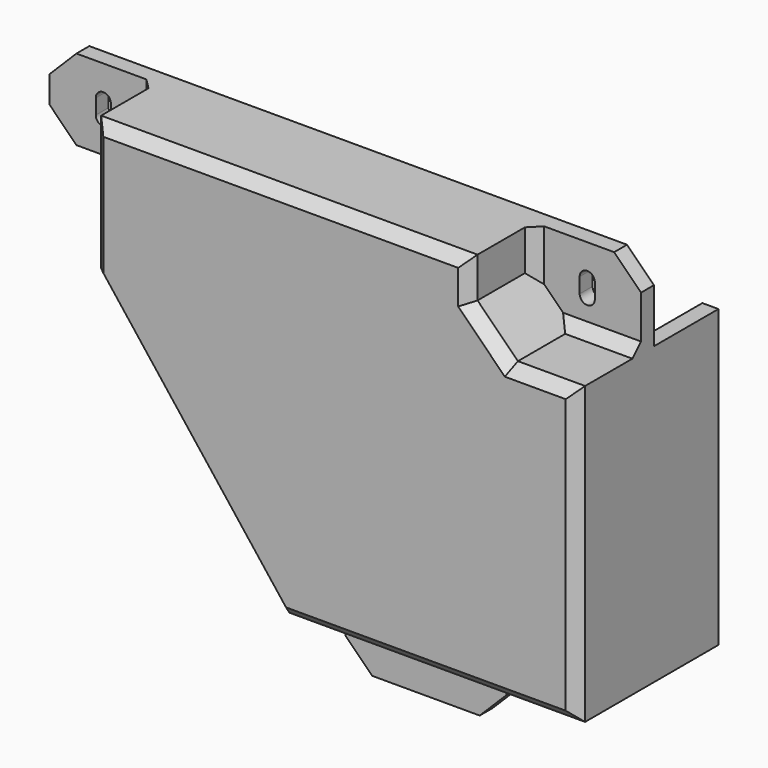
from build123d import *

# Parameters (mm, degrees)
F0_W      = 279.4
F0_H      = 213.36
F1_DEPTH  = 83.82
F2_W      = 76.2
F2_H      = 35.56
F2_W_2    = 50.8
F2_H_2    = 38.1
F3_DEPTH  = 38.1
F2_W_3    = 63.5
F4_DEPTH  = 83.82
F5_T      = -7.62
F6_W      = 38.1
F6_H      = 38.1
F6_H_2    = 35.56
F7_DEPTH  = 341.884
F9_DEPTH  = 7.62
F10_SIZE  = 5.08
F11_W     = 84.455
F11_H     = 38.1
F12_DEPTH = 25.4
F13_W     = 15.24
F13_H     = 12.7
F14_DEPTH = 12.7


# Not quite as in the source:
# - a feature names something its author has since deleted; it is built from what else it names


with BuildPart() as f1:
    # F0 (on Front) → F1 (new body)
    with BuildSketch(Plane.XZ):
        with Locations((-139.7, 106.68)):
            Rectangle(F0_W, F0_H)
    extrude(amount=F1_DEPTH)

    # F2 (on face) → F3 (cut)
    with BuildSketch(Plane.XZ.offset(83.82)):
        Polygon((0, 213.36), (-50.8, 213.36), (-50.8, 194.31), (-31.75, 175.26), (0, 175.26), align=None)
        with Locations((-101.6, 17.78)):
            Rectangle(F2_W, F2_H)
        with Locations((-254, 194.31)):
            Rectangle(F2_W_2, F2_H_2)
    extrude(amount=-F3_DEPTH, mode=Mode.SUBTRACT)

    # F2 (on face) → F4 (cut)
    with BuildSketch(Plane.XZ.offset(83.82)):
        Polygon((-228.6, 149.86), (-228.6, 175.26), (-279.4, 175.26), (-279.4, 0), (-139.7, 0), (-139.7, 35.56), align=None)
        with Locations((-31.75, 17.78)):
            Rectangle(F2_W_3, F2_H)
    extrude(amount=-F4_DEPTH, mode=Mode.SUBTRACT)

    # F5
    f5_openings = [f1.faces().sort_by_distance(p)[0] for p in [
        (-109.470638, 0, 127.051961),
    ]]
    offset(amount=F5_T, openings=f5_openings, kind=Kind.INTERSECTION)

    # F6 (on face) → F7 (cut)
    with BuildSketch(Plane.YZ):
        with Locations((-19.05, 194.31)):
            Rectangle(F6_W, F6_H)
        with Locations((-19.05, 17.78)):
            Rectangle(F6_W, F6_H_2)
    extrude(amount=-F7_DEPTH, mode=Mode.SUBTRACT)

    # F8 (on face) → F9 (cut)
    with BuildSketch(Plane.XZ.offset(45.72)):
        with BuildLine():
            ThreePointArc((-22.3094151415, 192.52565), (-21.9529005037, 193.3863524737), (-21.8313, 194.31))
            ThreePointArc((-21.8313, 194.31), (-21.9529005037, 195.2336475263), (-22.3094151415, 196.09435))
            ThreePointArc((-22.3094151415, 196.09435), (-23.61565, 194.7881151415), (-25.4, 194.31))
            ThreePointArc((-25.4, 194.31), (-23.61565, 193.8318848585), (-22.3094151415, 192.52565))
        make_face()
        with BuildLine():
            ThreePointArc((-25.4, 194.31), (-27.18435, 194.7881151415), (-28.4905848585, 196.09435))
            ThreePointArc((-28.4905848585, 196.09435), (-28.8470994963, 195.2336475263), (-28.9687, 194.31))
            ThreePointArc((-28.9687, 194.31), (-28.8470994963, 193.3863524737), (-28.4905848585, 192.52565))
            ThreePointArc((-28.4905848585, 192.52565), (-27.18435, 193.8318848585), (-25.4, 194.31))
        make_face()
        Polygon((0, 200.66), (0, 213.36), (-12.7, 213.36), align=None)
        with BuildLine():
            ThreePointArc((-250.9094151415, 192.52565), (-250.5529005037, 193.3863524737), (-250.4313, 194.31))
            ThreePointArc((-250.4313, 194.31), (-250.5529005037, 195.2336475263), (-250.9094151415, 196.09435))
            ThreePointArc((-250.9094151415, 196.09435), (-252.21565, 194.7881151415), (-254, 194.31))
            ThreePointArc((-254, 194.31), (-252.21565, 193.8318848585), (-250.9094151415, 192.52565))
        make_face()
        with BuildLine():
            ThreePointArc((-254, 194.31), (-255.78435, 194.7881151415), (-257.0905848585, 196.09435))
            ThreePointArc((-257.0905848585, 196.09435), (-257.4470994963, 195.2336475263), (-257.5687, 194.31))
            ThreePointArc((-257.5687, 194.31), (-257.4470994963, 193.3863524737), (-257.0905848585, 192.52565))
            ThreePointArc((-257.0905848585, 192.52565), (-255.78435, 193.8318848585), (-254, 194.31))
        make_face()
        Polygon((-279.4, 200.66), (-266.7, 213.36), (-279.4, 213.36), align=None)
        Polygon((-279.4, 175.26), (-266.7, 175.26), (-279.4, 187.96), align=None)
        Polygon((-127, 0), (-139.7, 12.7), (-139.7, 0), align=None)
        Polygon((-63.5, 12.7), (-76.2, 0), (-63.5, 0), align=None)
        with BuildLine():
            ThreePointArc((-82.55, 19.05), (-82.0714594891, 20.8359375), (-80.7640625, 22.1433344891))
            ThreePointArc((-80.7640625, 22.1433344891), (-81.6255307233, 22.5001663108), (-82.55, 22.621875))
            ThreePointArc((-82.55, 22.621875), (-83.4744692767, 22.5001663108), (-84.3359375, 22.1433344891))
            ThreePointArc((-84.3359375, 22.1433344891), (-83.0285405109, 20.8359375), (-82.55, 19.05))
        make_face()
        with BuildLine():
            ThreePointArc((-82.55, 15.478125), (-81.6255307233, 15.5998336892), (-80.7640625, 15.9566655109))
            ThreePointArc((-80.7640625, 15.9566655109), (-82.0714594891, 17.2640625), (-82.55, 19.05))
            ThreePointArc((-82.55, 19.05), (-83.0285405109, 17.2640625), (-84.3359375, 15.9566655109))
            ThreePointArc((-84.3359375, 15.9566655109), (-83.4744692767, 15.5998336892), (-82.55, 15.478125))
        make_face()
        with BuildLine():
            ThreePointArc((-120.65, 19.05), (-120.1714594891, 20.8359375), (-118.8640625, 22.1433344891))
            ThreePointArc((-118.8640625, 22.1433344891), (-119.7255307233, 22.5001663108), (-120.65, 22.621875))
            ThreePointArc((-120.65, 22.621875), (-121.5744692767, 22.5001663108), (-122.4359375, 22.1433344891))
            ThreePointArc((-122.4359375, 22.1433344891), (-121.1285405109, 20.8359375), (-120.65, 19.05))
        make_face()
        with BuildLine():
            ThreePointArc((-120.65, 15.478125), (-119.7255307233, 15.5998336892), (-118.8640625, 15.9566655109))
            ThreePointArc((-118.8640625, 15.9566655109), (-120.1714594891, 17.2640625), (-120.65, 19.05))
            ThreePointArc((-120.65, 19.05), (-121.1285405109, 17.2640625), (-122.4359375, 15.9566655109))
            ThreePointArc((-122.4359375, 15.9566655109), (-121.5744692767, 15.5998336892), (-120.65, 15.478125))
        make_face()
        with BuildLine():
            ThreePointArc((-28.4905848585, 196.09435), (-25.4, 197.8787), (-22.3094151415, 196.09435))
            ThreePointArc((-22.3094151415, 196.09435), (-21.9529005037, 196.9550524737), (-21.8313, 197.8787))
            ThreePointArc((-21.8313, 197.8787), (-25.4, 201.4474), (-28.9687, 197.8787))
            ThreePointArc((-28.9687, 197.8787), (-28.8470994963, 196.9550524737), (-28.4905848585, 196.09435))
        make_face()
        with BuildLine():
            ThreePointArc((-25.4, 194.31), (-23.61565, 194.7881151415), (-22.3094151415, 196.09435))
            ThreePointArc((-22.3094151415, 196.09435), (-25.4, 197.8787), (-28.4905848585, 196.09435))
            ThreePointArc((-28.4905848585, 196.09435), (-27.18435, 194.7881151415), (-25.4, 194.31))
        make_face()
        with BuildLine():
            ThreePointArc((-28.4905848585, 192.52565), (-25.4, 190.7413), (-22.3094151415, 192.52565))
            ThreePointArc((-22.3094151415, 192.52565), (-23.61565, 193.8318848585), (-25.4, 194.31))
            ThreePointArc((-25.4, 194.31), (-27.18435, 193.8318848585), (-28.4905848585, 192.52565))
        make_face()
        with BuildLine():
            ThreePointArc((-21.8313, 190.7413), (-21.9529005037, 191.6649475263), (-22.3094151415, 192.52565))
            ThreePointArc((-22.3094151415, 192.52565), (-25.4, 190.7413), (-28.4905848585, 192.52565))
            ThreePointArc((-28.4905848585, 192.52565), (-28.8470994963, 191.6649475263), (-28.9687, 190.7413))
            ThreePointArc((-28.9687, 190.7413), (-25.4, 187.1726), (-21.8313, 190.7413))
        make_face()
        with BuildLine():
            ThreePointArc((-28.9687, 194.31), (-28.8470994963, 195.2336475263), (-28.4905848585, 196.09435))
            ThreePointArc((-28.4905848585, 196.09435), (-28.8470994963, 196.9550524737), (-28.9687, 197.8787))
            Line((-28.9687, 197.8787), (-28.9687, 194.31))
        make_face()
        with BuildLine():
            ThreePointArc((-22.3094151415, 196.09435), (-21.9529005037, 195.2336475263), (-21.8313, 194.31))
            Line((-21.8313, 194.31), (-21.8313, 197.8787))
            ThreePointArc((-21.8313, 197.8787), (-21.9529005037, 196.9550524737), (-22.3094151415, 196.09435))
        make_face()
        with BuildLine():
            Line((-21.8313, 190.7413), (-21.8313, 194.31))
            ThreePointArc((-21.8313, 194.31), (-21.9529005037, 193.3863524737), (-22.3094151415, 192.52565))
            ThreePointArc((-22.3094151415, 192.52565), (-21.9529005037, 191.6649475263), (-21.8313, 190.7413))
        make_face()
        with BuildLine():
            ThreePointArc((-28.9687, 190.7413), (-28.8470994963, 191.6649475263), (-28.4905848585, 192.52565))
            ThreePointArc((-28.4905848585, 192.52565), (-28.8470994963, 193.3863524737), (-28.9687, 194.31))
            Line((-28.9687, 194.31), (-28.9687, 190.7413))
        make_face()
        with BuildLine():
            ThreePointArc((-122.4359375, 15.9566655109), (-121.1285405109, 17.2640625), (-120.65, 19.05))
            ThreePointArc((-120.65, 19.05), (-121.1285405109, 20.8359375), (-122.4359375, 22.1433344891))
            ThreePointArc((-122.4359375, 22.1433344891), (-124.221875, 19.05), (-122.4359375, 15.9566655109))
        make_face()
        with BuildLine():
            ThreePointArc((-118.8640625, 15.9566655109), (-117.5566655109, 17.2640625), (-117.078125, 19.05))
            ThreePointArc((-117.078125, 19.05), (-117.5566655109, 20.8359375), (-118.8640625, 22.1433344891))
            ThreePointArc((-118.8640625, 22.1433344891), (-120.1714594891, 20.8359375), (-120.65, 19.05))
            ThreePointArc((-120.65, 19.05), (-120.1714594891, 17.2640625), (-118.8640625, 15.9566655109))
        make_face()
        with BuildLine():
            ThreePointArc((-118.8640625, 22.1433344891), (-117.5566655109, 20.8359375), (-117.078125, 19.05))
            ThreePointArc((-117.078125, 19.05), (-117.5566655109, 17.2640625), (-118.8640625, 15.9566655109))
            ThreePointArc((-118.8640625, 15.9566655109), (-118.0025942767, 15.5998336892), (-117.078125, 15.478125))
            ThreePointArc((-117.078125, 15.478125), (-114.5524279659, 16.5243029659), (-113.50625, 19.05))
            ThreePointArc((-113.50625, 19.05), (-114.5524279659, 21.5756970341), (-117.078125, 22.621875))
            ThreePointArc((-117.078125, 22.621875), (-118.0025942767, 22.5001663108), (-118.8640625, 22.1433344891))
        make_face()
        with BuildLine():
            ThreePointArc((-122.4359375, 15.9566655109), (-124.221875, 19.05), (-122.4359375, 22.1433344891))
            ThreePointArc((-122.4359375, 22.1433344891), (-123.2974057233, 22.5001663108), (-124.221875, 22.621875))
            ThreePointArc((-124.221875, 22.621875), (-127.79375, 19.05), (-124.221875, 15.478125))
            ThreePointArc((-124.221875, 15.478125), (-123.2974057233, 15.5998336892), (-122.4359375, 15.9566655109))
        make_face()
        with BuildLine():
            ThreePointArc((-120.65, 22.621875), (-119.7255307233, 22.5001663108), (-118.8640625, 22.1433344891))
            ThreePointArc((-118.8640625, 22.1433344891), (-118.0025942767, 22.5001663108), (-117.078125, 22.621875))
            Line((-117.078125, 22.621875), (-120.65, 22.621875))
        make_face()
        with BuildLine():
            ThreePointArc((-122.4359375, 22.1433344891), (-121.5744692767, 22.5001663108), (-120.65, 22.621875))
            Line((-120.65, 22.621875), (-124.221875, 22.621875))
            ThreePointArc((-124.221875, 22.621875), (-123.2974057233, 22.5001663108), (-122.4359375, 22.1433344891))
        make_face()
        with BuildLine():
            ThreePointArc((-117.078125, 15.478125), (-118.0025942767, 15.5998336892), (-118.8640625, 15.9566655109))
            ThreePointArc((-118.8640625, 15.9566655109), (-119.7255307233, 15.5998336892), (-120.65, 15.478125))
            Line((-120.65, 15.478125), (-117.078125, 15.478125))
        make_face()
        with BuildLine():
            Line((-124.221875, 15.478125), (-120.65, 15.478125))
            ThreePointArc((-120.65, 15.478125), (-121.5744692767, 15.5998336892), (-122.4359375, 15.9566655109))
            ThreePointArc((-122.4359375, 15.9566655109), (-123.2974057233, 15.5998336892), (-124.221875, 15.478125))
        make_face()
        with BuildLine():
            ThreePointArc((-82.55, 22.621875), (-81.6255307233, 22.5001663108), (-80.7640625, 22.1433344891))
            ThreePointArc((-80.7640625, 22.1433344891), (-79.9025942767, 22.5001663108), (-78.978125, 22.621875))
            Line((-78.978125, 22.621875), (-82.55, 22.621875))
        make_face()
        with BuildLine():
            ThreePointArc((-84.3359375, 22.1433344891), (-83.4744692767, 22.5001663108), (-82.55, 22.621875))
            Line((-82.55, 22.621875), (-86.121875, 22.621875))
            ThreePointArc((-86.121875, 22.621875), (-85.1974057233, 22.5001663108), (-84.3359375, 22.1433344891))
        make_face()
        with BuildLine():
            ThreePointArc((-84.3359375, 15.9566655109), (-86.121875, 19.05), (-84.3359375, 22.1433344891))
            ThreePointArc((-84.3359375, 22.1433344891), (-85.1974057233, 22.5001663108), (-86.121875, 22.621875))
            ThreePointArc((-86.121875, 22.621875), (-89.69375, 19.05), (-86.121875, 15.478125))
            ThreePointArc((-86.121875, 15.478125), (-85.1974057233, 15.5998336892), (-84.3359375, 15.9566655109))
        make_face()
        with BuildLine():
            ThreePointArc((-84.3359375, 15.9566655109), (-83.0285405109, 17.2640625), (-82.55, 19.05))
            ThreePointArc((-82.55, 19.05), (-83.0285405109, 20.8359375), (-84.3359375, 22.1433344891))
            ThreePointArc((-84.3359375, 22.1433344891), (-86.121875, 19.05), (-84.3359375, 15.9566655109))
        make_face()
        with BuildLine():
            ThreePointArc((-80.7640625, 15.9566655109), (-79.4566655109, 17.2640625), (-78.978125, 19.05))
            ThreePointArc((-78.978125, 19.05), (-79.4566655109, 20.8359375), (-80.7640625, 22.1433344891))
            ThreePointArc((-80.7640625, 22.1433344891), (-82.0714594891, 20.8359375), (-82.55, 19.05))
            ThreePointArc((-82.55, 19.05), (-82.0714594891, 17.2640625), (-80.7640625, 15.9566655109))
        make_face()
        with BuildLine():
            ThreePointArc((-80.7640625, 22.1433344891), (-79.4566655109, 20.8359375), (-78.978125, 19.05))
            ThreePointArc((-78.978125, 19.05), (-79.4566655109, 17.2640625), (-80.7640625, 15.9566655109))
            ThreePointArc((-80.7640625, 15.9566655109), (-79.9025942767, 15.5998336892), (-78.978125, 15.478125))
            ThreePointArc((-78.978125, 15.478125), (-76.4524279659, 16.5243029659), (-75.40625, 19.05))
            ThreePointArc((-75.40625, 19.05), (-76.4524279659, 21.5756970341), (-78.978125, 22.621875))
            ThreePointArc((-78.978125, 22.621875), (-79.9025942767, 22.5001663108), (-80.7640625, 22.1433344891))
        make_face()
        with BuildLine():
            ThreePointArc((-78.978125, 15.478125), (-79.9025942767, 15.5998336892), (-80.7640625, 15.9566655109))
            ThreePointArc((-80.7640625, 15.9566655109), (-81.6255307233, 15.5998336892), (-82.55, 15.478125))
            Line((-82.55, 15.478125), (-78.978125, 15.478125))
        make_face()
        with BuildLine():
            Line((-86.121875, 15.478125), (-82.55, 15.478125))
            ThreePointArc((-82.55, 15.478125), (-83.4744692767, 15.5998336892), (-84.3359375, 15.9566655109))
            ThreePointArc((-84.3359375, 15.9566655109), (-85.1974057233, 15.5998336892), (-86.121875, 15.478125))
        make_face()
        with BuildLine():
            ThreePointArc((-254, 194.31), (-252.21565, 194.7881151415), (-250.9094151415, 196.09435))
            ThreePointArc((-250.9094151415, 196.09435), (-254, 197.8787), (-257.0905848585, 196.09435))
            ThreePointArc((-257.0905848585, 196.09435), (-255.78435, 194.7881151415), (-254, 194.31))
        make_face()
        with BuildLine():
            ThreePointArc((-257.0905848585, 196.09435), (-254, 197.8787), (-250.9094151415, 196.09435))
            ThreePointArc((-250.9094151415, 196.09435), (-250.5529005037, 196.9550524737), (-250.4313, 197.8787))
            ThreePointArc((-250.4313, 197.8787), (-254, 201.4474), (-257.5687, 197.8787))
            ThreePointArc((-257.5687, 197.8787), (-257.4470994963, 196.9550524737), (-257.0905848585, 196.09435))
        make_face()
        with BuildLine():
            ThreePointArc((-257.0905848585, 192.52565), (-254, 190.7413), (-250.9094151415, 192.52565))
            ThreePointArc((-250.9094151415, 192.52565), (-252.21565, 193.8318848585), (-254, 194.31))
            ThreePointArc((-254, 194.31), (-255.78435, 193.8318848585), (-257.0905848585, 192.52565))
        make_face()
        with BuildLine():
            ThreePointArc((-250.4313, 190.7413), (-250.5529005037, 191.6649475263), (-250.9094151415, 192.52565))
            ThreePointArc((-250.9094151415, 192.52565), (-254, 190.7413), (-257.0905848585, 192.52565))
            ThreePointArc((-257.0905848585, 192.52565), (-257.4470994963, 191.6649475263), (-257.5687, 190.7413))
            ThreePointArc((-257.5687, 190.7413), (-254, 187.1726), (-250.4313, 190.7413))
        make_face()
        with BuildLine():
            Line((-250.4313, 190.7413), (-250.4313, 194.31))
            ThreePointArc((-250.4313, 194.31), (-250.5529005037, 193.3863524737), (-250.9094151415, 192.52565))
            ThreePointArc((-250.9094151415, 192.52565), (-250.5529005037, 191.6649475263), (-250.4313, 190.7413))
        make_face()
        with BuildLine():
            ThreePointArc((-250.9094151415, 196.09435), (-250.5529005037, 195.2336475263), (-250.4313, 194.31))
            Line((-250.4313, 194.31), (-250.4313, 197.8787))
            ThreePointArc((-250.4313, 197.8787), (-250.5529005037, 196.9550524737), (-250.9094151415, 196.09435))
        make_face()
        with BuildLine():
            ThreePointArc((-257.5687, 194.31), (-257.4470994963, 195.2336475263), (-257.0905848585, 196.09435))
            ThreePointArc((-257.0905848585, 196.09435), (-257.4470994963, 196.9550524737), (-257.5687, 197.8787))
            Line((-257.5687, 197.8787), (-257.5687, 194.31))
        make_face()
        with BuildLine():
            ThreePointArc((-257.5687, 190.7413), (-257.4470994963, 191.6649475263), (-257.0905848585, 192.52565))
            ThreePointArc((-257.0905848585, 192.52565), (-257.4470994963, 193.3863524737), (-257.5687, 194.31))
            Line((-257.5687, 194.31), (-257.5687, 190.7413))
        make_face()
    extrude(amount=-F9_DEPTH, mode=Mode.SUBTRACT)

    # F10
    f10_edges = [f1.edges().sort_by_distance(p)[0] for p in [
        (-50.8, -45.72, 203.835),
        (-15.875, -45.72, 175.26),
        (-228.6, -45.72, 194.31),
        (-101.6, -45.72, 35.56),
        (-220.98, -76.2, 179.107241),
        (-139.7, -76.2, 205.74),
        (-58.42, -76.2, 198.446846),
        (-46.663154, -76.2, 179.396846),
        (-21.263154, -76.2, 167.64),
        (-7.62, -76.2, 105.41),
        (-71.796591, -76.2, 43.18),
        (-178.476591, -76.2, 97.827241),
        (-139.7, -83.82, 213.36),
        (-228.6, -83.82, 181.61),
        (-184.15, -83.82, 92.71),
        (-69.85, -83.82, 35.56),
        (0, -83.82, 105.41),
        (-15.875, -83.82, 175.26),
        (-41.275, -83.82, 184.785),
        (-50.8, -83.82, 203.835),
    ]]
    chamfer(f10_edges, length=F10_SIZE)

    # F11 (on face) → F12 (cut)
    with BuildSketch(Plane(origin=(0, 0, 35.56), x_dir=(1, 0, 0), z_dir=(0, 0, -1))):
        Polygon((-71.12, 38.1), (-71.12, 0), (-50.8, 0), (-50.8, 38.1), (-63.5, 38.1), align=None)
        with Locations((-113.3475, 19.05)):
            Rectangle(F11_W, F11_H)
    extrude(amount=-F12_DEPTH, mode=Mode.SUBTRACT)

    # F13 (on face) → F14 (join)
    with BuildSketch(Plane(origin=(0, -76.2, 0), x_dir=(-1, 0, 0), z_dir=(0, 1, 0))):
        with Locations((134.62, 156.21)):
            Rectangle(F13_W, F13_H)
        with Locations((134.62, 74.93)):
            Rectangle(F13_W, F13_H)
    extrude(amount=F14_DEPTH)


solid = f1.part
